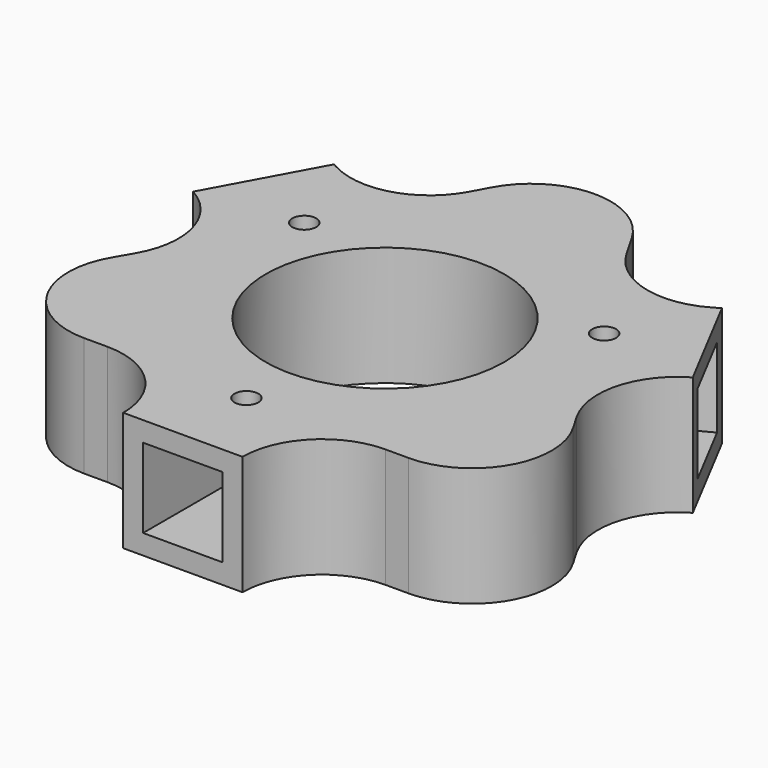
from build123d import *

# Parameters (mm, degrees)
F0_R     = 1.5
F0_R_2   = 15
F1_DEPTH = 15
F2_W     = 10
F2_H     = 10
F3_DEPTH = 15
F4_W     = 10
F4_H     = 10
F5_DEPTH = 15
F6_W     = 10
F6_H     = 10
F7_DEPTH = 15
F8_R     = 9.99999


# Not quite as in the source:
# - a fillet or chamfer is up to 0.001 mm smaller than in the source, because OpenCascade refuses the exact size


with BuildPart() as f1:
    # F0 (on Top) → F1 (new body)
    with BuildSketch(Plane.XY):
        Polygon((-24.3407530135, 22.4126278684), (-31.5135795584, 9.2387689289), (-22.7389262459, 4.1727204769), (-37.7220713048, -21.7788480222), (-7.5, -21.7788480222), (-7.5, -31.7788480222), (0, -31.7788480222), (7.5, -31.7788480222), (7.5, -21.7788480222), (37.7220713048, -21.7788480222), (22.8180813967, 4.0356197342), (31.4860692862, 9.0400848755), (24.5212116355, 22.3250672958), (14.9900065464, 16.8222234719), (-0.6591394661, 43.9273394607), (-15.1098627306, 17.3866460996), align=None)
        with Locations((0, -21.7788480222)):
            Circle(F0_R, mode=Mode.SUBTRACT)
        Circle(F0_R_2, mode=Mode.SUBTRACT)
        with Locations((-18.8610356524, 10.8894240111)):
            Circle(F0_R, mode=Mode.SUBTRACT)
        with Locations((18.8610356524, 10.8894240111)):
            Circle(F0_R, mode=Mode.SUBTRACT)
    extrude(amount=F1_DEPTH)

    # F2 (on face) → F3 (cut)
    with BuildSketch(Plane.XZ.offset(31.7788480222)):
        with Locations((0, 7.5)):
            Rectangle(F2_W, F2_H)
    extrude(amount=-F3_DEPTH, mode=Mode.SUBTRACT)

    # F4 (on face) → F5 (cut)
    with BuildSketch(Plane(origin=(-28.1875812899, 15.3474112818, 0), x_dir=(-0.4781884363, -0.8782572626, 0), z_dir=(-0.8782572626, 0.4781884363, 0))):
        with Locations((0, 7.5)):
            Rectangle(F4_W, F4_H)
    extrude(amount=-F5_DEPTH, mode=Mode.SUBTRACT)

    # F6 (on face) → F7 (cut)
    with BuildSketch(Plane(origin=(28.415383594, 14.8972046453, 0), x_dir=(-0.4643238434, 0.8856654947, 0), z_dir=(0.8856654947, 0.4643238434, 0))):
        with Locations((0.8867585393, 7.5)):
            Rectangle(F6_W, F6_H)
    extrude(amount=-F7_DEPTH, mode=Mode.SUBTRACT)

    # F8 (radius 10 in the source; OpenCascade refuses exactly that, so slightly less here)
    f8_edges = [f1.edges().sort_by_distance(p)[0] for p in [
        (37.722071, -21.778848, 7.5),
        (-0.659139, 43.927339, 7.5),
        (14.990007, 16.822223, 7.5),
        (22.818081, 4.03562, 7.5),
        (7.5, -21.778848, 7.5),
        (-7.5, -21.778848, 7.5),
        (-37.722071, -21.778848, 7.5),
        (-22.738926, 4.17272, 7.5),
        (-15.109863, 17.386646, 7.5),
    ]]
    fillet(f8_edges, radius=F8_R)


solid = f1.part
